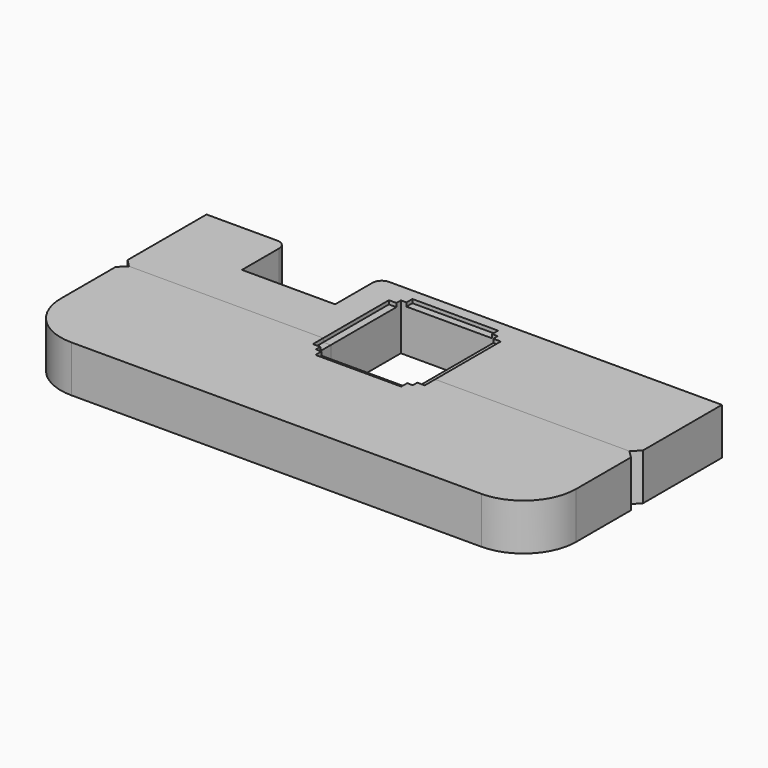
from build123d import *

# Parameters (mm, degrees)
F0_W      = 6.604
F0_H      = 2.54
F1_DEPTH  = 6.35
F0_H_2    = 1.27
F0_W_2    = 2.54
F2_DEPTH  = 6.35
F3_DEPTH  = 2.032
F6_DEPTH  = 5.08
F7_DEPTH  = 24.13
F8_DEPTH  = 14.478
F11_W     = 1.016
F11_H     = 1.778
F12_DEPTH = 0.508
F13_DEPTH = 0.508
F14_R     = 1.27


# Not quite as in the source:
# - a feature names something its author has since deleted; it is built from what else it names


with BuildPart() as f1:
    # F0 (on Top) → F1 (new body)
    with BuildSketch(Plane.XY):
        Polygon((-9.144, -14.478), (-9.144, 0), (-11.4935, 0), (-11.4935, -7.62), (-24.1935, -7.62), (-24.1935, 0), (-35.1155, 0), (-35.1155, -13.462), (-34.0995, -14.478), align=None)
        Polygon((35.1155, 0), (9.144, 0), (9.144, -14.478), (34.0995, -14.478), (35.1155, -13.462), align=None)
        Polygon((-6.604, -2.54), (-6.604, 0), (-9.144, 0), (-9.144, -14.478), (-6.604, -14.478), align=None)
        with Locations((-3.302, -1.27)):
            Rectangle(F0_W, F0_H)
        Polygon((9.144, 0), (0, 0), (0, -2.54), (6.604, -2.54), (6.604, -14.478), (9.144, -14.478), align=None)
    extrude(amount=F1_DEPTH)

    # F5 (on face) + F4 (on face) → F6 (cut)
    with BuildSketch(Plane(origin=(0, 0, 0), x_dir=(-1, 0, 0), z_dir=(0, 1, 0))):
        with BuildLine():
            ThreePointArc((-29.1465, 3.175), (-31.9405, 5.969), (-34.7345, 3.175))
            Line((-34.7345, 3.175), (-33.3375, 3.175))
            ThreePointArc((-33.3375, 3.175), (-31.9405, 4.572), (-30.5435, 3.175))
            Line((-30.5435, 3.175), (-29.1465, 3.175))
        make_face()
        with BuildLine():
            Line((-33.3375, 3.175), (-34.7345, 3.175))
            ThreePointArc((-34.7345, 3.175), (-31.9405, 0.381), (-29.1465, 3.175))
            Line((-29.1465, 3.175), (-30.5435, 3.175))
            ThreePointArc((-30.5435, 3.175), (-31.9405, 1.778), (-33.3375, 3.175))
        make_face()
        with BuildLine():
            Line((-33.2105, 3.175), (-33.3375, 3.175))
            ThreePointArc((-33.3375, 3.175), (-31.9405, 1.778), (-30.5435, 3.175))
            Line((-30.5435, 3.175), (-30.6705, 3.175))
            ThreePointArc((-30.6705, 3.175), (-31.9405, 1.905), (-33.2105, 3.175))
        make_face()
        with BuildLine():
            Line((-30.6705, 3.175), (-33.2105, 3.175))
            ThreePointArc((-33.2105, 3.175), (-31.9405, 1.905), (-30.6705, 3.175))
        make_face()
        with BuildLine():
            ThreePointArc((-30.5435, 3.175), (-31.9405, 4.572), (-33.3375, 3.175))
            Line((-33.3375, 3.175), (-33.2105, 3.175))
            ThreePointArc((-33.2105, 3.175), (-31.9405, 4.445), (-30.6705, 3.175))
            Line((-30.6705, 3.175), (-30.5435, 3.175))
        make_face()
        with BuildLine():
            ThreePointArc((-30.6705, 3.175), (-31.9405, 4.445), (-33.2105, 3.175))
            Line((-33.2105, 3.175), (-30.6705, 3.175))
        make_face()
    with BuildSketch(Plane(origin=(0, 0, 0), x_dir=(-1, 0, 0), z_dir=(0, 1, 0))):
        with BuildLine():
            Line((33.3375, 3.175), (34.7345, 3.175))
            ThreePointArc((34.7345, 3.175), (31.9405, 5.969), (29.1465, 3.175))
            Line((29.1465, 3.175), (30.5435, 3.175))
            ThreePointArc((30.5435, 3.175), (31.9405, 4.572), (33.3375, 3.175))
        make_face()
        with BuildLine():
            ThreePointArc((29.1465, 3.175), (31.9405, 0.381), (34.7345, 3.175))
            Line((34.7345, 3.175), (33.3375, 3.175))
            ThreePointArc((33.3375, 3.175), (31.9405, 1.778), (30.5435, 3.175))
            Line((30.5435, 3.175), (29.1465, 3.175))
        make_face()
        with BuildLine():
            ThreePointArc((30.5435, 3.175), (31.9405, 1.778), (33.3375, 3.175))
            Line((33.3375, 3.175), (33.2105, 3.175))
            ThreePointArc((33.2105, 3.175), (31.9405, 1.905), (30.6705, 3.175))
            Line((30.6705, 3.175), (30.5435, 3.175))
        make_face()
        with BuildLine():
            Line((33.2105, 3.175), (33.3375, 3.175))
            ThreePointArc((33.3375, 3.175), (31.9405, 4.572), (30.5435, 3.175))
            Line((30.5435, 3.175), (30.6705, 3.175))
            ThreePointArc((30.6705, 3.175), (31.9405, 4.445), (33.2105, 3.175))
        make_face()
        with BuildLine():
            Line((30.6705, 3.175), (33.2105, 3.175))
            ThreePointArc((33.2105, 3.175), (31.9405, 4.445), (30.6705, 3.175))
        make_face()
        with BuildLine():
            ThreePointArc((30.6705, 3.175), (31.9405, 1.905), (33.2105, 3.175))
            Line((33.2105, 3.175), (30.6705, 3.175))
        make_face()
    extrude(amount=-F6_DEPTH, mode=Mode.SUBTRACT)


with BuildPart() as f2:
    # F0 (on Top) → F2 (new body)
    with BuildSketch(Plane.XY):
        with BuildLine():
            ThreePointArc((-20.7645, -24.8285), (-27.94, -17.653), (-35.1155, -24.8285))
            ThreePointArc((-35.1155, -24.8285), (-33.0138447084, -29.9023447084), (-27.94, -32.004))
            ThreePointArc((-27.94, -32.004), (-22.8661552916, -29.9023447084), (-20.7645, -24.8285))
        make_face()
        with BuildLine():
            ThreePointArc((27.94, -32.004), (33.0138447084, -29.9023447084), (35.1155, -24.8285))
            ThreePointArc((35.1155, -24.8285), (22.8661552916, -19.7546552916), (27.94, -32.004))
        make_face()
        with Locations((-3.302, -17.653)):
            Rectangle(F0_W, F0_H_2)
        with BuildLine():
            Line((-9.144, -19.558), (-9.144, -14.478))
            Line((-9.144, -14.478), (-34.0995, -14.478))
            Line((-34.0995, -14.478), (-35.1155, -15.494))
            Line((-35.1155, -15.494), (-35.1155, -24.8285))
            ThreePointArc((-35.1155, -24.8285), (-27.94, -17.653), (-20.7645, -24.8285))
            ThreePointArc((-20.7645, -24.8285), (-22.8661552916, -29.9023447084), (-27.94, -32.004))
            Line((-27.94, -32.004), (0, -32.004))
            Line((0, -32.004), (0, -19.558))
            Line((0, -19.558), (-9.144, -19.558))
        make_face()
        Polygon((9.144, -19.558), (9.144, -17.018), (6.604, -17.018), (6.604, -18.288), (6.604, -19.558), align=None)
        with Locations((7.874, -15.748)):
            Rectangle(F0_W_2, F0_H)
        with Locations((3.302, -18.923)):
            Rectangle(F0_W, F0_H_2)
        with BuildLine():
            Line((34.0995, -14.478), (9.144, -14.478))
            Line((9.144, -14.478), (9.144, -17.018))
            Line((9.144, -17.018), (9.144, -19.558))
            Line((9.144, -19.558), (6.604, -19.558))
            Line((6.604, -19.558), (0, -19.558))
            Line((0, -19.558), (0, -32.004))
            Line((0, -32.004), (27.94, -32.004))
            ThreePointArc((27.94, -32.004), (22.8661552916, -19.7546552916), (35.1155, -24.8285))
            Line((35.1155, -24.8285), (35.1155, -15.494))
            Line((35.1155, -15.494), (34.0995, -14.478))
        make_face()
        Polygon((-6.604, -14.478), (-9.144, -14.478), (-9.144, -19.558), (0, -19.558), (0, -18.288), (-6.604, -18.288), (-6.604, -17.018), align=None)
        with Locations((3.302, -17.653)):
            Rectangle(F0_W, F0_H_2)
    extrude(amount=F2_DEPTH)

    # F0 (on Top) → F3 (cut)
    with BuildSketch(Plane.XY):
        with Locations((3.302, -17.653)):
            Rectangle(F0_W, F0_H_2)
        with Locations((-3.302, -17.653)):
            Rectangle(F0_W, F0_H_2)
    extrude(amount=F3_DEPTH, mode=Mode.SUBTRACT)


with BuildPart() as f7_tool:
    # F5 (on face) + F4 (on face) → F7 (new body)
    with BuildSketch(Plane(origin=(0, 0, 0), x_dir=(-1, 0, 0), z_dir=(0, 1, 0))):
        with BuildLine():
            ThreePointArc((-30.6705, 3.175), (-31.9405, 4.445), (-33.2105, 3.175))
            Line((-33.2105, 3.175), (-30.6705, 3.175))
        make_face()
        with BuildLine():
            Line((-30.6705, 3.175), (-33.2105, 3.175))
            ThreePointArc((-33.2105, 3.175), (-31.9405, 1.905), (-30.6705, 3.175))
        make_face()
    with BuildSketch(Plane(origin=(0, 0, 0), x_dir=(-1, 0, 0), z_dir=(0, 1, 0))):
        with BuildLine():
            Line((30.6705, 3.175), (33.2105, 3.175))
            ThreePointArc((33.2105, 3.175), (31.9405, 4.445), (30.6705, 3.175))
        make_face()
        with BuildLine():
            ThreePointArc((30.6705, 3.175), (31.9405, 1.905), (33.2105, 3.175))
            Line((33.2105, 3.175), (30.6705, 3.175))
        make_face()
    extrude(amount=-F7_DEPTH)


with BuildPart() as f1_1:
    add(f1.part)

    # F7: cut by f7_tool
    add(f7_tool.part, mode=Mode.SUBTRACT)

    # F5 (on face) + F4 (on face) → F8 (cut, through all)
    with BuildSketch(Plane(origin=(0, 0, 0), x_dir=(-1, 0, 0), z_dir=(0, 1, 0))):
        with BuildLine():
            ThreePointArc((-30.5435, 3.175), (-31.9405, 4.572), (-33.3375, 3.175))
            Line((-33.3375, 3.175), (-33.2105, 3.175))
            ThreePointArc((-33.2105, 3.175), (-31.9405, 4.445), (-30.6705, 3.175))
            Line((-30.6705, 3.175), (-30.5435, 3.175))
        make_face()
        with BuildLine():
            Line((-33.2105, 3.175), (-33.3375, 3.175))
            ThreePointArc((-33.3375, 3.175), (-31.9405, 1.778), (-30.5435, 3.175))
            Line((-30.5435, 3.175), (-30.6705, 3.175))
            ThreePointArc((-30.6705, 3.175), (-31.9405, 1.905), (-33.2105, 3.175))
        make_face()
    with BuildSketch(Plane(origin=(0, 0, 0), x_dir=(-1, 0, 0), z_dir=(0, 1, 0))):
        with BuildLine():
            Line((30.6705, 3.175), (33.2105, 3.175))
            ThreePointArc((33.2105, 3.175), (31.9405, 4.445), (30.6705, 3.175))
        make_face()
        with BuildLine():
            ThreePointArc((30.6705, 3.175), (31.9405, 1.905), (33.2105, 3.175))
            Line((33.2105, 3.175), (30.6705, 3.175))
        make_face()
    extrude(amount=-F8_DEPTH, mode=Mode.SUBTRACT)


with BuildPart() as f2_1:
    add(f2.part)

    # F7: cut by f7_tool
    add(f7_tool.part, mode=Mode.SUBTRACT)


with BuildPart() as f12_tool:
    # F9 (on face) + F10 (on face) + F11 (on face) → F12 (new body)
    with BuildSketch(Plane.XY.offset(6.35)):
        Polygon((-5.842, -2.54), (0, -2.54), (5.842, -2.54), (5.842, -1.524), (-5.842, -1.524), align=None)
    with BuildSketch(Plane.XY.offset(6.35)):
        Polygon((5.842, -18.034), (5.842, -17.018), (0, -17.018), (-5.842, -17.018), (-5.842, -18.034), align=None)
    with BuildSketch(Plane.XY.offset(6.35)):
        with Locations((-7.112, -15.367)):
            Rectangle(F11_W, F11_H)
        with Locations((7.112, -15.367)):
            Rectangle(F11_W, F11_H)
    extrude(amount=-F12_DEPTH)


with BuildPart() as f1_2:
    add(f1_1.part)

    # F12: cut by f12_tool
    add(f12_tool.part, mode=Mode.SUBTRACT)

    # F11 (on face) → F13 (cut)
    with BuildSketch(Plane.XY.offset(6.35)):
        Polygon((-6.604, -14.478), (-6.604, -9.779), (-6.604, -3.302), (-7.62, -3.302), (-7.62, -14.478), align=None)
        Polygon((6.604, -3.302), (6.604, -9.779), (6.604, -14.478), (7.62, -14.478), (7.62, -3.302), align=None)
    extrude(amount=-F13_DEPTH, mode=Mode.SUBTRACT)

    # F14
    f14_edges = [f1_2.edges().sort_by_distance(p)[0] for p in [
        (-11.4935, 0, 3.175),
        (-24.1935, 0, 3.175),
    ]]
    fillet(f14_edges, radius=F14_R)


with BuildPart() as f2_2:
    add(f2_1.part)

    # F12: cut by f12_tool
    add(f12_tool.part, mode=Mode.SUBTRACT)


solid = Compound([f1_2.part, f2_2.part])
